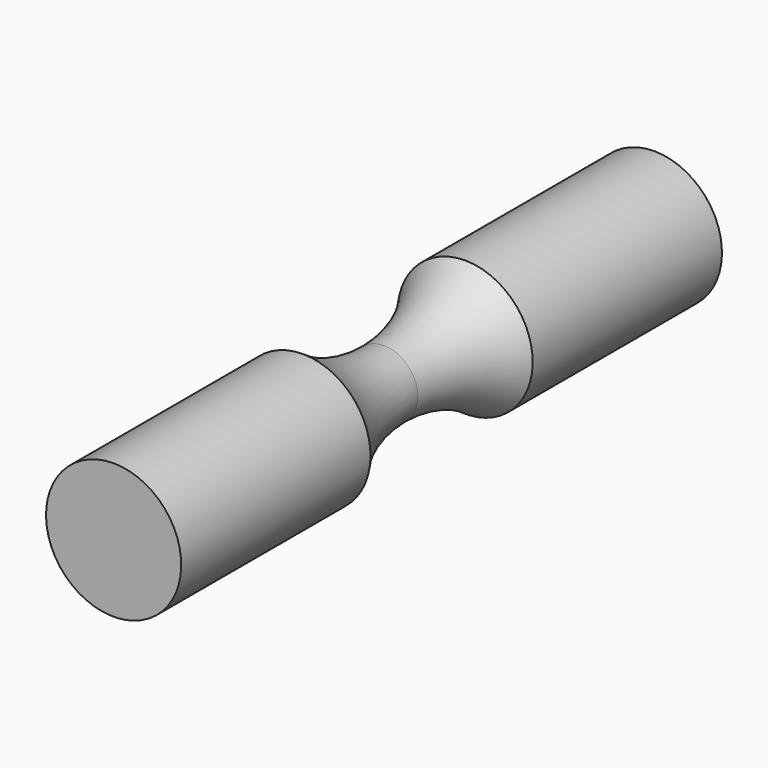
from build123d import *
from build123d import SkipClean  # not in build123d's __all__


with BuildPart() as f1:
    # F0 (on Right) → F1 (revolve)
    with BuildSketch(Plane.YZ):
        with BuildLine():
            Line((-30, 20), (-100, 20))
            Line((-100, 20), (-100, 0))
            Line((-100, 0), (0, 0))
            Line((0, 0), (0, 10))
            ThreePointArc((0, 10), (-15.8113883008, 12.5658350975), (-30, 20))
        make_face()
    revolve(axis=Axis((0, -50, 0), (0, 1, 0)))

    # F2: F1 across plane


with BuildPart() as f1_1:
    add(f1.part, clean=False)
    with SkipClean():  # cleaning this boolean's faces spoils the solid; the shape is the same uncleaned
        add(f1.part.mirror(Plane.XZ), clean=False)


solid = f1_1.part
